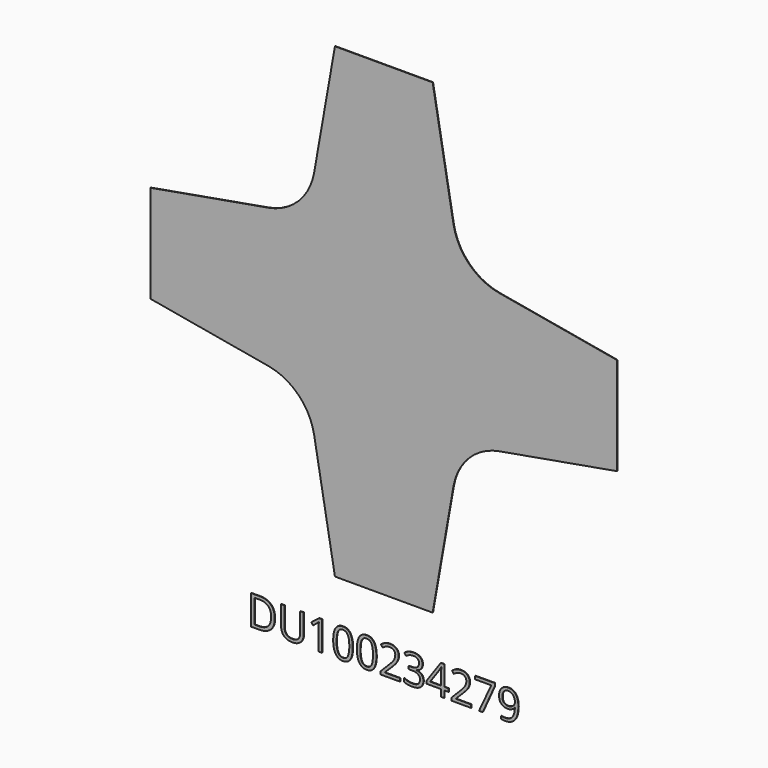
from build123d import *

# Parameters (mm, degrees)
F0_TEXT_SIZE = 42.8237020969
F1_DEPTH     = 0.508


# Not quite as in the source:
# - Text() gives the source's letters only with a copy of the font that has no kerning and outlines rounded to 1/6400 em; it was checked with that copy


with BuildPart() as f1:
    # F0 (on Front) → F1 (new body)
    with BuildSketch(Plane.XZ):
        with BuildLine():
            ThreePointArc((-72.007531069, 119.3954734607), (-88.2308218431, 88.2308218431), (-119.3954734607, 72.007531069))
            Line((-119.3954734607, 72.007531069), (-79.1108050234, 79.1108050234))
            Line((-79.1108050234, 79.1108050234), (-72.007531069, 119.3954734607))
        make_face()
        Polygon((-79.1108050234, 79.1108050234), (-119.3954734607, 72.007531069), (-241.3, 50.5124739697), (-241.3, 0), (-241.3, -50.5124739697), (-119.3954734607, -72.007531069), (-79.1108050234, -79.1108050234), (-72.007531069, -119.3954734607), (-50.5124739697, -241.3), (0, -241.3), (50.5124739697, -241.3), (72.007531069, -119.3954734607), (79.1108050234, -79.1108050234), (119.3954734607, -72.007531069), (241.3, -50.5124739697), (241.3, 0), (241.3, 50.5124739697), (119.3954734607, 72.007531069), (79.1108050234, 79.1108050234), (72.007531069, 119.3954734607), (50.5124739697, 241.3), (0, 241.3), (-50.5124739697, 241.3), (-72.007531069, 119.3954734607), align=None)
        with BuildLine():
            Line((-79.1108050234, -79.1108050234), (-119.3954734607, -72.007531069))
            ThreePointArc((-119.3954734607, -72.007531069), (-88.2308218431, -88.2308218431), (-72.007531069, -119.3954734607))
            Line((-72.007531069, -119.3954734607), (-79.1108050234, -79.1108050234))
        make_face()
        with BuildLine():
            ThreePointArc((119.3954734607, 72.007531069), (88.2308218431, 88.2308218431), (72.007531069, 119.3954734607))
            Line((72.007531069, 119.3954734607), (79.1108050234, 79.1108050234))
            Line((79.1108050234, 79.1108050234), (119.3954734607, 72.007531069))
        make_face()
        with BuildLine():
            Line((79.1108050234, -79.1108050234), (72.007531069, -119.3954734607))
            ThreePointArc((72.007531069, -119.3954734607), (88.2308218431, -88.2308218431), (119.3954734607, -72.007531069))
            Line((119.3954734607, -72.007531069), (79.1108050234, -79.1108050234))
        make_face()
        with Locations((-141.3393765688, -315.101057291)):
            Text('DU100234279', F0_TEXT_SIZE, font='Open Sans', text_align=(TextAlign.LEFT, TextAlign.BOTTOM))
    extrude(amount=F1_DEPTH)


solid = f1.part
